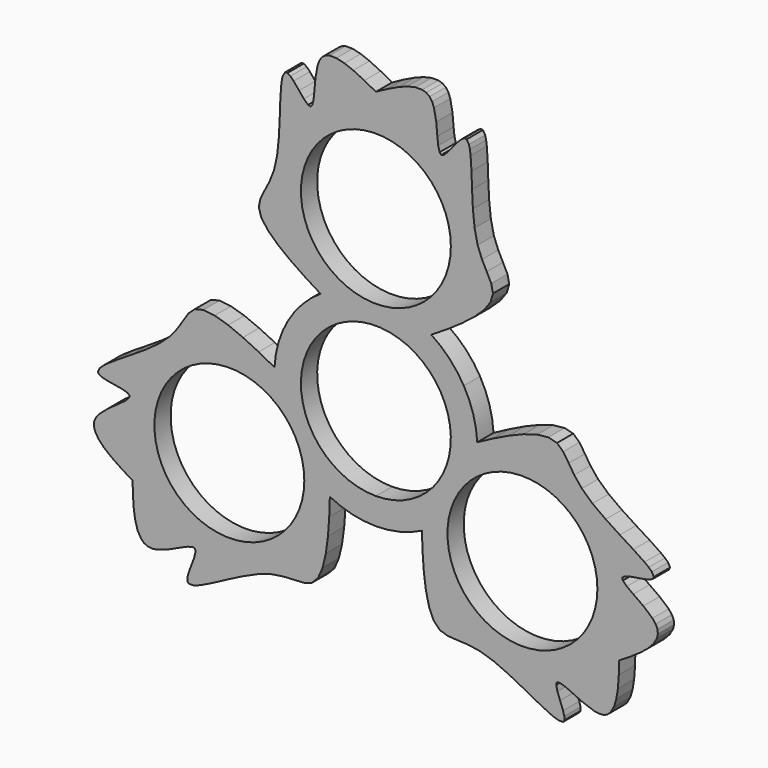
from build123d import *

# Parameters (mm, degrees)
F0_R     = 11.075
F1_DEPTH = 3


# Not quite as in the source:
# - ends of sketch curves that miss each other by under 0.0002 mm in the source are joined


with BuildPart() as f1:
    # F0 (on Front) → F1 (new body)
    with BuildSketch(Plane.XZ):
        with BuildLine():
            Line((1.697006, 36.15958), (0, 35.242249))
            Line((0, 35.242249), (-1.697006, 36.15958))
            Line((-1.697006, 36.15958), (-3.336401, 36.949437))
            Line((-3.336401, 36.949437), (-4.63887, 37.448648))
            Line((-4.63887, 37.448648), (-5.822377, 37.729185))
            Line((-5.822377, 37.729185), (-6.851356, 37.732795))
            Line((-6.851356, 37.732795), (-7.436324, 37.551423))
            Line((-7.436324, 37.551423), (-7.92537, 37.20226))
            Line((-7.92537, 37.20226), (-8.308095, 36.66842))
            Line((-8.308095, 36.66842), (-8.586956, 35.960699))
            Line((-8.586956, 35.960699), (-8.91576, 34.223652))
            Line((-8.91576, 34.223652), (-9.083737, 32.405421))
            Line((-9.083737, 32.405421), (-9.208416, 31.239412))
            Line((-9.208416, 31.239412), (-9.413198, 30.438367))
            Line((-9.413198, 30.438367), (-9.663329, 30.182956))
            Line((-9.663329, 30.182956), (-10.023812, 30.286843))
            Line((-10.023812, 30.286843), (-10.638429, 30.862092))
            Line((-10.638429, 30.862092), (-11.344187, 31.712131))
            Line((-11.344187, 31.712131), (-12.153084, 32.689686))
            Line((-12.153084, 32.689686), (-12.633154, 33.1756))
            Line((-12.633154, 33.1756), (-13.054918, 33.450628))
            Line((-13.054918, 33.450628), (-13.41268, 33.421971))
            Line((-13.41268, 33.421971), (-13.745343, 32.876595))
            Line((-13.745343, 32.876595), (-13.890056, 32.27158))
            Line((-13.890056, 32.27158), (-13.994393, 31.497866))
            Line((-13.994393, 31.497866), (-14.123195, 29.507511))
            Line((-14.123195, 29.507511), (-14.208532, 27.154252))
            Line((-14.208532, 27.154252), (-14.334094, 24.666091))
            Line((-14.334094, 24.666091), (-14.583569, 22.271026))
            Line((-14.583569, 22.271026), (-15.038601, 20.194187))
            Line((-15.038601, 20.194187), (-15.685996, 18.527616))
            Line((-15.685996, 18.527616), (-16.379707, 17.176927))
            Line((-16.379707, 17.176927), (-17.039503, 15.855872))
            Line((-17.039503, 15.855872), (-17.302388, 14.645365))
            Line((-17.302388, 14.645365), (-16.940362, 13.38409))
            Line((-16.940362, 13.38409), (-15.944051, 12.029363))
            Line((-15.944051, 12.029363), (-14.440514, 10.612535))
            Line((-14.440514, 10.612535), (-12.558887, 9.166081))
            Line((-12.558887, 9.166081), (-10.428306, 7.722477))
            Line((-10.428306, 7.722477), (-8.177905, 6.314198))
            ThreePointArc((-8.177905, 6.314198), (-10.8840298531, 4.0612655348), (-12.9903810426, 1.2395460246))
            ThreePointArc((-12.9903810426, 1.2395460246), (-14.3808861682, -1.9954671282), (-14.9789204431, -5.4655059765))
            Line((-14.9789204431, -5.4655059765), (-17.323726, -4.220742))
            Line((-17.323726, -4.220742), (-19.639215, -3.097406))
            Line((-19.639215, -3.097406), (-21.832694, -2.191097))
            Line((-21.832694, -2.191097), (-23.811472, -1.597409))
            Line((-23.811472, -1.597409), (-25.482855, -1.411942))
            Line((-25.482855, -1.411942), (-26.756164, -1.729056))
            Line((-26.756164, -1.729056), (-27.673052, -2.561975))
            Line((-27.673052, -2.561975), (-28.487221, -3.793902))
            Line((-28.487221, -3.793902), (-29.310096, -5.070018))
            Line((-29.310096, -5.070018), (-30.429692, -6.463964))
            Line((-30.429692, -6.463964), (-32.000771, -7.896453))
            Line((-32.000771, -7.896453), (-33.95022, -9.310037))
            Line((-33.95022, -9.310037), (-36.042251, -10.662857))
            Line((-36.042251, -10.662857), (-38.037564, -11.91339))
            Line((-38.037564, -11.91339), (-39.696861, -13.020114))
            Line((-39.696861, -13.020114), (-40.314749, -13.49733))
            Line((-40.314749, -13.49733), (-40.76635, -13.925162))
            Line((-40.76635, -13.925162), (-41.072328, -14.485945))
            Line((-41.072328, -14.485945), (-40.918265, -14.810105))
            Line((-40.918265, -14.810105), (-40.469201, -15.037848))
            Line((-40.469201, -15.037848), (-39.808353, -15.210645))
            Line((-39.808353, -15.210645), (-38.557317, -15.422392))
            Line((-38.557317, -15.422392), (-37.468282, -15.608577))
            Line((-37.468282, -15.608577), (-36.662794, -15.853227))
            Line((-36.662794, -15.853227), (-36.392584, -16.11347))
            Line((-36.392584, -16.11347), (-36.48871, -16.457795))
            Line((-36.48871, -16.457795), (-37.080044, -17.035665))
            Line((-37.080044, -17.035665), (-38.027499, -17.726644))
            Line((-38.027499, -17.726644), (-39.518144, -18.781233))
            Line((-39.518144, -18.781233), (-40.858069, -19.934509))
            Line((-40.858069, -19.934509), (-41.331542, -20.52987))
            Line((-41.331542, -20.52987), (-41.602499, -21.128239))
            Line((-41.602499, -21.128239), (-41.660361, -21.726347))
            Line((-41.660361, -21.726347), (-41.524949, -22.32363))
            Line((-41.524949, -22.32363), (-41.007333, -23.212947))
            Line((-41.007333, -23.212947), (-40.172628, -24.097626))
            Line((-40.172628, -24.097626), (-39.089064, -24.975991))
            Line((-39.089064, -24.975991), (-37.58533, -26.00082))
            Line((-37.58533, -26.00082), (-35.942395, -27.011805))
            Line((-35.942395, -27.011805), (-35.888324, -28.940121))
            Line((-35.888324, -28.940121), (-35.752663, -30.754808))
            Line((-35.752663, -30.754808), (-35.533758, -32.132384))
            Line((-35.533758, -32.132384), (-35.184956, -33.297599))
            Line((-35.184956, -33.297599), (-34.673593, -34.190526))
            Line((-34.673593, -34.190526), (-34.224037, -34.606438))
            Line((-34.224037, -34.606438), (-33.677129, -34.855383))
            Line((-33.677129, -34.855383), (-33.023448, -34.919912))
            Line((-33.023448, -34.919912), (-32.271113, -34.807552))
            Line((-32.271113, -34.807552), (-30.602384, -34.223781))
            Line((-30.602384, -34.223781), (-28.943761, -33.460139))
            Line((-28.943761, -33.460139), (-27.871629, -32.985109))
            Line((-27.871629, -32.985109), (-27.075512, -32.761933))
            Line((-27.075512, -32.761933), (-26.729255, -32.850848))
            Line((-26.729255, -32.850848), (-26.638982, -33.214979))
            Line((-26.638982, -33.214979), (-26.829854, -34.034877))
            Line((-26.829854, -34.034877), (-27.21313, -35.0711))
            Line((-27.21313, -35.0711), (-27.655269, -36.260404))
            Line((-27.655269, -36.260404), (-27.836047, -36.919114))
            Line((-27.836047, -36.919114), (-27.863347, -37.421885))
            Line((-27.863347, -37.421885), (-27.659648, -37.717388))
            Line((-27.659648, -37.717388), (-27.021007, -37.732795))
            Line((-27.021007, -37.732795), (-26.424693, -37.555613))
            Line((-26.424693, -37.555613), (-25.702468, -37.259114))
            Line((-25.702468, -37.259114), (-23.914368, -36.375482))
            Line((-23.914368, -36.375482), (-21.833718, -35.272757))
            Line((-21.833718, -35.272757), (-19.616127, -34.137416))
            Line((-19.616127, -34.137416), (-17.417202, -33.155935))
            Line((-17.417202, -33.155935), (-15.39109, -32.511585))
            Line((-15.39109, -32.511585), (-13.6241, -32.23896))
            Line((-13.6241, -32.23896), (-12.107514, -32.164387))
            Line((-12.107514, -32.164387), (-10.633549, -32.07526))
            Line((-10.633549, -32.07526), (-9.453776, -31.697671))
            Line((-9.453776, -31.697671), (-8.542493, -30.75351))
            Line((-8.542493, -30.75351), (-7.867421, -29.213316))
            Line((-7.867421, -29.213316), (-7.39218, -27.202801))
            Line((-7.39218, -27.202801), (-7.080328, -24.850037))
            Line((-7.080328, -24.850037), (-6.89542, -22.283097))
            Line((-6.89542, -22.283097), (-6.801015, -19.630054))
            ThreePointArc((-6.801015, -19.630054), (-3.4968560233, -20.8471602064), (0, -21.260454))
            ThreePointArc((0, -21.260454), (3.4968560233, -20.8471602064), (6.8010148611, -19.630053727))
            Line((6.8010148611, -19.630053727), (6.89542, -22.283097))
            Line((6.89542, -22.283097), (7.080328, -24.850037))
            Line((7.080328, -24.850037), (7.39218, -27.202801))
            Line((7.39218, -27.202801), (7.867421, -29.213316))
            Line((7.867421, -29.213316), (8.542493, -30.75351))
            Line((8.542493, -30.75351), (9.453776, -31.697671))
            Line((9.453776, -31.697671), (10.633549, -32.07526))
            Line((10.633549, -32.07526), (12.107514, -32.164387))
            Line((12.107514, -32.164387), (13.6241, -32.23896))
            Line((13.6241, -32.23896), (15.39109, -32.511585))
            Line((15.39109, -32.511585), (17.417202, -33.155935))
            Line((17.417202, -33.155935), (19.616127, -34.137416))
            Line((19.616127, -34.137416), (21.833718, -35.272757))
            Line((21.833718, -35.272757), (23.914368, -36.375482))
            Line((23.914368, -36.375482), (25.702468, -37.259114))
            Line((25.702468, -37.259114), (26.424693, -37.555613))
            Line((26.424693, -37.555613), (27.021007, -37.732795))
            Line((27.021007, -37.732795), (27.659648, -37.717388))
            Line((27.659648, -37.717388), (27.863347, -37.421885))
            Line((27.863347, -37.421885), (27.836047, -36.919114))
            Line((27.836047, -36.919114), (27.655269, -36.260404))
            Line((27.655269, -36.260404), (27.21313, -35.0711))
            Line((27.21313, -35.0711), (26.829854, -34.034877))
            Line((26.829854, -34.034877), (26.638982, -33.214979))
            Line((26.638982, -33.214979), (26.729255, -32.850848))
            Line((26.729255, -32.850848), (27.075512, -32.761933))
            Line((27.075512, -32.761933), (27.871629, -32.985109))
            Line((27.871629, -32.985109), (28.943761, -33.460139))
            Line((28.943761, -33.460139), (30.602384, -34.223781))
            Line((30.602384, -34.223781), (32.271113, -34.807552))
            Line((32.271113, -34.807552), (33.023448, -34.919912))
            Line((33.023448, -34.919912), (33.677129, -34.855383))
            Line((33.677129, -34.855383), (34.224037, -34.606438))
            Line((34.224037, -34.606438), (34.673593, -34.190526))
            Line((34.673593, -34.190526), (35.184956, -33.297599))
            Line((35.184956, -33.297599), (35.533758, -32.132384))
            Line((35.533758, -32.132384), (35.752663, -30.754808))
            Line((35.752663, -30.754808), (35.888324, -28.940121))
            Line((35.888324, -28.940121), (35.942395, -27.011805))
            Line((35.942395, -27.011805), (37.58533, -26.00082))
            Line((37.58533, -26.00082), (39.089064, -24.975991))
            Line((39.089064, -24.975991), (40.172628, -24.097626))
            Line((40.172628, -24.097626), (41.007333, -23.212947))
            Line((41.007333, -23.212947), (41.524949, -22.32363))
            Line((41.524949, -22.32363), (41.660361, -21.726347))
            Line((41.660361, -21.726347), (41.602499, -21.128239))
            Line((41.602499, -21.128239), (41.331542, -20.52987))
            Line((41.331542, -20.52987), (40.858069, -19.934509))
            Line((40.858069, -19.934509), (39.518144, -18.781233))
            Line((39.518144, -18.781233), (38.027499, -17.726644))
            Line((38.027499, -17.726644), (37.080044, -17.035665))
            Line((37.080044, -17.035665), (36.48871, -16.457795))
            Line((36.48871, -16.457795), (36.392584, -16.11347))
            Line((36.392584, -16.11347), (36.662794, -15.853227))
            Line((36.662794, -15.853227), (37.468282, -15.608577))
            Line((37.468282, -15.608577), (38.557317, -15.422392))
            Line((38.557317, -15.422392), (39.808353, -15.210645))
            Line((39.808353, -15.210645), (40.469201, -15.037848))
            Line((40.469201, -15.037848), (40.918265, -14.810105))
            Line((40.918265, -14.810105), (41.072328, -14.485945))
            Line((41.072328, -14.485945), (40.76635, -13.925162))
            Line((40.76635, -13.925162), (40.314749, -13.49733))
            Line((40.314749, -13.49733), (39.696861, -13.020114))
            Line((39.696861, -13.020114), (38.037564, -11.91339))
            Line((38.037564, -11.91339), (36.042251, -10.662857))
            Line((36.042251, -10.662857), (33.95022, -9.310037))
            Line((33.95022, -9.310037), (32.000771, -7.896453))
            Line((32.000771, -7.896453), (30.429692, -6.463964))
            Line((30.429692, -6.463964), (29.310096, -5.070018))
            Line((29.310096, -5.070018), (28.487221, -3.793902))
            Line((28.487221, -3.793902), (27.673052, -2.561975))
            Line((27.673052, -2.561975), (26.756164, -1.729056))
            Line((26.756164, -1.729056), (25.482855, -1.411942))
            Line((25.482855, -1.411942), (23.811472, -1.597409))
            Line((23.811472, -1.597409), (21.832694, -2.191097))
            Line((21.832694, -2.191097), (19.639215, -3.097406))
            Line((19.639215, -3.097406), (17.323726, -4.220742))
            Line((17.323726, -4.220742), (14.97892, -5.465506))
            ThreePointArc((14.97892, -5.465506), (14.3808861682, -1.9954671282), (12.9903810426, 1.2395460246))
            ThreePointArc((12.9903810426, 1.2395460246), (10.8840298531, 4.0612655348), (8.1779049435, 6.3141979131))
            Line((8.1779049435, 6.3141979131), (10.428306, 7.722477))
            Line((10.428306, 7.722477), (12.558887, 9.166081))
            Line((12.558887, 9.166081), (14.440514, 10.612535))
            Line((14.440514, 10.612535), (15.944051, 12.029363))
            Line((15.944051, 12.029363), (16.940362, 13.38409))
            Line((16.940362, 13.38409), (17.302388, 14.645365))
            Line((17.302388, 14.645365), (17.039503, 15.855872))
            Line((17.039503, 15.855872), (16.379707, 17.176927))
            Line((16.379707, 17.176927), (15.685996, 18.527616))
            Line((15.685996, 18.527616), (15.038601, 20.194187))
            Line((15.038601, 20.194187), (14.583569, 22.271026))
            Line((14.583569, 22.271026), (14.334094, 24.666091))
            Line((14.334094, 24.666091), (14.208532, 27.154252))
            Line((14.208532, 27.154252), (14.123195, 29.507511))
            Line((14.123195, 29.507511), (13.994393, 31.497866))
            Line((13.994393, 31.497866), (13.890056, 32.27158))
            Line((13.890056, 32.27158), (13.745343, 32.876595))
            Line((13.745343, 32.876595), (13.41268, 33.421971))
            Line((13.41268, 33.421971), (13.054918, 33.450628))
            Line((13.054918, 33.450628), (12.633154, 33.1756))
            Line((12.633154, 33.1756), (12.153084, 32.689686))
            Line((12.153084, 32.689686), (11.344187, 31.712131))
            Line((11.344187, 31.712131), (10.638429, 30.862092))
            Line((10.638429, 30.862092), (10.023812, 30.286843))
            Line((10.023812, 30.286843), (9.663329, 30.182956))
            Line((9.663329, 30.182956), (9.413198, 30.438367))
            Line((9.413198, 30.438367), (9.208416, 31.239412))
            Line((9.208416, 31.239412), (9.083737, 32.405421))
            Line((9.083737, 32.405421), (8.91576, 34.223652))
            Line((8.91576, 34.223652), (8.586956, 35.960699))
            Line((8.586956, 35.960699), (8.308095, 36.66842))
            Line((8.308095, 36.66842), (7.92537, 37.20226))
            Line((7.92537, 37.20226), (7.436324, 37.551423))
            Line((7.436324, 37.551423), (6.851356, 37.732795))
            Line((6.851356, 37.732795), (5.822377, 37.729185))
            Line((5.822377, 37.729185), (4.63887, 37.448648))
            Line((4.63887, 37.448648), (3.336401, 36.949437))
            Line((3.336401, 36.949437), (1.697006, 36.15958))
        make_face()
        with Locations((-21.650635, -18.760454)):
            Circle(F0_R, mode=Mode.SUBTRACT)
        with BuildLine():
            ThreePointArc((9.5912312602, -0.7229538498), (9.5912313903, -11.7979539249), (0, -17.335454))
            ThreePointArc((0, -17.335454), (-9.5912313903, -11.7979539249), (-9.5912312602, -0.7229538498))
            ThreePointArc((-9.5912312602, -0.7229538498), (0, 4.814546), (9.5912312602, -0.7229538498))
        make_face(mode=Mode.SUBTRACT)
        with Locations((21.650635, -18.760454)):
            Circle(F0_R, mode=Mode.SUBTRACT)
        with Locations((0, 18.739546)):
            Circle(F0_R, mode=Mode.SUBTRACT)
    extrude(amount=F1_DEPTH)


solid = f1.part
